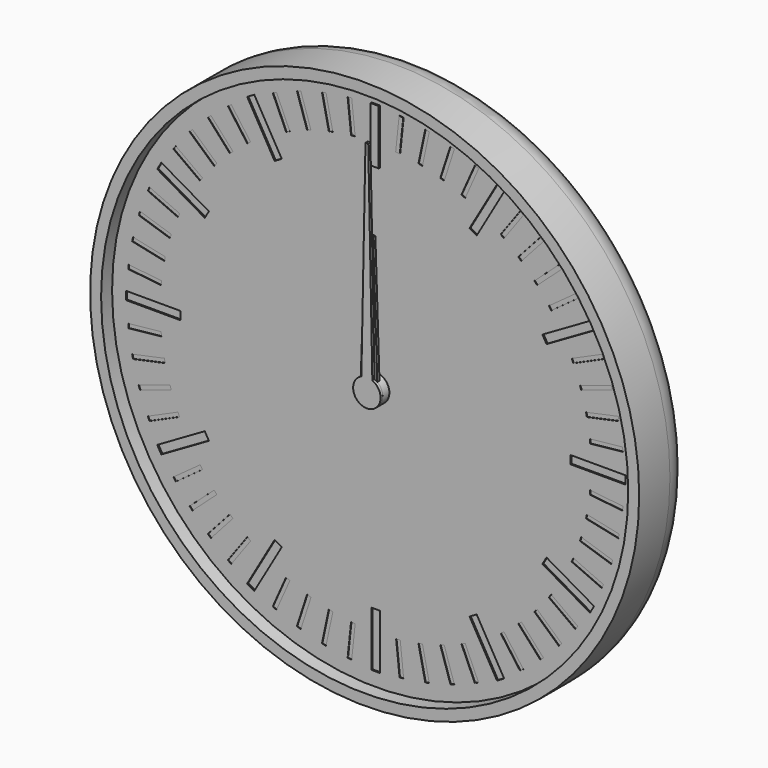
from build123d import *

# Parameters (mm, degrees)
F0_R      = 100
F1_DEPTH  = 24
F2_R      = 10
F3_T      = -4
F4_R      = 5
F4_R_2    = 3
F5_DEPTH  = 2
F6_DEPTH  = 19
F7_DEPTH  = 8
F9_DEPTH  = 4
F11_DEPTH = 4
F12_R     = 5
F12_R_2   = 3
F13_DEPTH = 2
F14_R     = 3
F15_DEPTH = 4
F17_DEPTH = 4
F18_R     = 3
F19_DEPTH = 2
F20_R     = 98
F20_R_2   = 5
F21_DEPTH = 1
F23_R     = 5
F23_R_2   = 3
F24_DEPTH = 2
F25_W     = 3
F25_H     = 20
F25_W_2   = 20
F25_H_2   = 3
F26_DEPTH = 0.5
F27_W     = 1.5
F27_H     = 12
F27_W_2   = 12
F27_H_2   = 1.5
F28_DEPTH = 0.2
F29_DEPTH = 1
F30_DEPTH = 0.4
F31_R     = 5
F31_R_2   = 3
F32_DEPTH = 5
F33_R     = 3
F34_DEPTH = 1
F36_DEPTH = 1


with BuildPart() as f1:
    # F0 (on Front) → F1 (new body)
    with BuildSketch(Plane.XZ):
        Circle(F0_R)
    extrude(amount=F1_DEPTH)

    # F2
    f2_edges = [f1.edges().sort_by_distance(p)[0] for p in [
        (-100, 0, 0),
    ]]
    fillet(f2_edges, radius=F2_R)

    # F3
    f3_openings = [f1.faces().sort_by_distance(p)[0] for p in [
        (0, -24, 0),
    ]]
    offset(amount=F3_T, openings=f3_openings)

    # F4 (on face) → F5 (join)
    with BuildSketch(Plane.XZ.offset(4)):
        Circle(F4_R)
        Circle(F4_R_2, mode=Mode.SUBTRACT)
        with Locations((40, 0)):
            Circle(F4_R)
        with Locations((40, 0)):
            Circle(F4_R_2, mode=Mode.SUBTRACT)
    extrude(amount=F5_DEPTH)


with BuildPart() as f6:
    # F6 (new): a face of the model
    f6_faces = [f1.part.faces().sort_by_distance(p)[0] for p in [
        (0, -4, 0),
    ]]
    extrude(f6_faces, amount=F6_DEPTH)

    # F8 (on face) → F9 (join)
    with BuildSketch(Plane.XZ.offset(6)):
        with BuildLine():
            ThreePointArc((9.2729637667, -1.3794085621), (9.3494561423, -0.6915886375), (9.375, 0))
            ThreePointArc((9.375, 0), (9.3494561423, 0.6915886375), (9.2729637667, 1.3794085621))
            ThreePointArc((9.2729637667, 1.3794085621), (8.9161548403, 2.8970343223), (8.3127812852, 4.3345463782))
            ThreePointArc((8.3127812852, 4.3345463782), (7.5845343223, 5.5104867402), (6.6911892658, 6.566476316))
            ThreePointArc((6.6911892658, 6.566476316), (5.5104867402, 7.5845343223), (4.1773988938, 8.3928519278))
            ThreePointArc((4.1773988938, 8.3928519278), (2.8970343223, 8.9161548403), (1.5536078905, 9.2453733036))
            ThreePointArc((1.5536078905, 9.2453733036), (0, 9.375), (-1.5536078905, 9.2453733036))
            ThreePointArc((-1.5536078905, 9.2453733036), (-2.8970343223, 8.9161548403), (-4.1773988938, 8.3928519278))
            ThreePointArc((-4.1773988938, 8.3928519278), (-5.5104867402, 7.5845343223), (-6.6911892658, 6.566476316))
            ThreePointArc((-6.6911892658, 6.566476316), (-7.5845343223, 5.5104867402), (-8.3127812852, 4.3345463782))
            ThreePointArc((-8.3127812852, 4.3345463782), (-8.9161548403, 2.8970343223), (-9.2729637667, 1.3794085621))
            ThreePointArc((-9.2729637667, 1.3794085621), (-9.375, 0), (-9.2729637667, -1.3794085621))
            ThreePointArc((-9.2729637667, -1.3794085621), (-8.9161548403, -2.8970343223), (-8.3127812852, -4.3345463782))
            ThreePointArc((-8.3127812852, -4.3345463782), (-7.5845343223, -5.5104867402), (-6.6911892658, -6.566476316))
            ThreePointArc((-6.6911892658, -6.566476316), (-5.5104867402, -7.5845343223), (-4.1773988938, -8.3928519278))
            ThreePointArc((-4.1773988938, -8.3928519278), (-2.8970343223, -8.9161548403), (-1.5536078905, -9.2453733036))
            ThreePointArc((-1.5536078905, -9.2453733036), (0, -9.375), (1.5536078905, -9.2453733036))
            ThreePointArc((1.5536078905, -9.2453733036), (2.8970343223, -8.9161548403), (4.1773988938, -8.3928519278))
            ThreePointArc((4.1773988938, -8.3928519278), (5.5104867402, -7.5845343223), (6.6911892658, -6.566476316))
            ThreePointArc((6.6911892658, -6.566476316), (7.5845343223, -5.5104867402), (8.3127812852, -4.3345463782))
            ThreePointArc((8.3127812852, -4.3345463782), (8.9161548403, -2.8970343223), (9.2729637667, -1.3794085621))
        make_face()
        with BuildLine():
            ThreePointArc((8.3127812852, 4.3345463782), (8.9161548403, 2.8970343223), (9.2729637667, 1.3794085621))
            Line((9.2729637667, 1.3794085621), (11.1823199426, 2.3946312492))
            Line((11.1823199426, 2.3946312492), (10.8182678729, 3.515068311))
            Line((10.8182678729, 3.515068311), (10.4542158031, 4.6355053728))
            Line((10.4542158031, 4.6355053728), (8.3127812852, 4.3345463782))
        make_face()
        with BuildLine():
            Line((11.1823199426, -2.3946312492), (9.2729637667, -1.3794085621))
            ThreePointArc((9.2729637667, -1.3794085621), (8.9161548403, -2.8970343223), (8.3127812852, -4.3345463782))
            Line((8.3127812852, -4.3345463782), (10.4542158031, -4.6355053728))
            Line((10.4542158031, -4.6355053728), (10.8182678729, -3.515068311))
            Line((10.8182678729, -3.515068311), (11.1823199426, -2.3946312492))
        make_face()
        with BuildLine():
            ThreePointArc((4.1773988938, 8.3928519278), (5.5104867402, 7.5845343223), (6.6911892658, 6.566476316))
            Line((6.6911892658, 6.566476316), (7.6391579371, 8.5101001246))
            Line((7.6391579371, 8.5101001246), (6.6860572448, 9.202568311))
            Line((6.6860572448, 9.202568311), (5.7329565525, 9.8950364974))
            Line((5.7329565525, 9.8950364974), (4.1773988938, 8.3928519278))
        make_face()
        with BuildLine():
            Line((7.6391579371, -8.5101001246), (6.6911892658, -6.566476316))
            ThreePointArc((6.6911892658, -6.566476316), (5.5104867402, -7.5845343223), (4.1773988938, -8.3928519278))
            Line((4.1773988938, -8.3928519278), (5.7329565525, -9.8950364974))
            Line((5.7329565525, -9.8950364974), (6.6860572448, -9.202568311))
            Line((6.6860572448, -9.202568311), (7.6391579371, -8.5101001246))
        make_face()
        with BuildLine():
            ThreePointArc((-1.5536078905, 9.2453733036), (0, 9.375), (1.5536078905, 9.2453733036))
            Line((1.5536078905, 9.2453733036), (1.1780972451, 11.375))
            Line((1.1780972451, 11.375), (0, 11.375))
            Line((0, 11.375), (-1.1780972451, 11.375))
            Line((-1.1780972451, 11.375), (-1.5536078905, 9.2453733036))
        make_face()
        with BuildLine():
            Line((1.1780972451, -11.375), (1.5536078905, -9.2453733036))
            ThreePointArc((1.5536078905, -9.2453733036), (0, -9.375), (-1.5536078905, -9.2453733036))
            Line((-1.5536078905, -9.2453733036), (-1.1780972451, -11.375))
            Line((-1.1780972451, -11.375), (0, -11.375))
            Line((0, -11.375), (1.1780972451, -11.375))
        make_face()
        with BuildLine():
            ThreePointArc((-6.6911892658, 6.566476316), (-5.5104867402, 7.5845343223), (-4.1773988938, 8.3928519278))
            Line((-4.1773988938, 8.3928519278), (-5.7329565525, 9.8950364974))
            Line((-5.7329565525, 9.8950364974), (-6.6860572448, 9.202568311))
            Line((-6.6860572448, 9.202568311), (-7.6391579371, 8.5101001246))
            Line((-7.6391579371, 8.5101001246), (-6.6911892658, 6.566476316))
        make_face()
        with BuildLine():
            Line((-5.7329565525, -9.8950364974), (-4.1773988938, -8.3928519278))
            ThreePointArc((-4.1773988938, -8.3928519278), (-5.5104867402, -7.5845343223), (-6.6911892658, -6.566476316))
            Line((-6.6911892658, -6.566476316), (-7.6391579371, -8.5101001246))
            Line((-7.6391579371, -8.5101001246), (-6.6860572448, -9.202568311))
            Line((-6.6860572448, -9.202568311), (-5.7329565525, -9.8950364974))
        make_face()
        with BuildLine():
            ThreePointArc((-9.2729637667, 1.3794085621), (-8.9161548403, 2.8970343223), (-8.3127812852, 4.3345463782))
            Line((-8.3127812852, 4.3345463782), (-10.4542158031, 4.6355053728))
            Line((-10.4542158031, 4.6355053728), (-10.8182678729, 3.515068311))
            Line((-10.8182678729, 3.515068311), (-11.1823199426, 2.3946312492))
            Line((-11.1823199426, 2.3946312492), (-9.2729637667, 1.3794085621))
        make_face()
        with BuildLine():
            Line((-10.4542158031, -4.6355053728), (-8.3127812852, -4.3345463782))
            ThreePointArc((-8.3127812852, -4.3345463782), (-8.9161548403, -2.8970343223), (-9.2729637667, -1.3794085621))
            Line((-9.2729637667, -1.3794085621), (-11.1823199426, -2.3946312492))
            Line((-11.1823199426, -2.3946312492), (-10.8182678729, -3.515068311))
            Line((-10.8182678729, -3.515068311), (-10.4542158031, -4.6355053728))
        make_face()
    extrude(amount=F9_DEPTH)

    # F35 (on face) → F36 (join)
    with BuildSketch(Plane.XZ.offset(23)):
        with BuildLine():
            ThreePointArc((-2, 4.582575695), (-2.7386127875, -4.1833001327), (5, 0))
            ThreePointArc((5, 0), (4.1833001327, 2.7386127875), (2, 4.582575695))
            ThreePointArc((2, 4.582575695), (0, 5), (-2, 4.582575695))
        make_face()
        with BuildLine():
            ThreePointArc((-2, 4.582575695), (0, 5), (2, 4.582575695))
            Line((2, 4.582575695), (0.5, 80))
            Line((0.5, 80), (0, 80))
            Line((0, 80), (-0.5, 80))
            Line((-0.5, 80), (-2, 4.582575695))
        make_face()
    extrude(amount=-F36_DEPTH)


with BuildPart() as f7:
    # F7 (new): a face of the model
    f7_faces = [f1.part.faces().sort_by_distance(p)[0] for p in [
        (40, -4, 0),
    ]]
    extrude(f7_faces, amount=F7_DEPTH)

    # F10 (on face) → F11 (join)
    with BuildSketch(Plane.XZ.offset(6)):
        with BuildLine():
            ThreePointArc((68.0829066802, -1.5381733945), (68.1144747006, -0.7693746225), (68.125, 0))
            ThreePointArc((68.125, 0), (68.1144747006, 0.7693746225), (68.0829066802, 1.5381733945))
            ThreePointArc((68.0829066802, 1.5381733945), (67.9709283072, 2.9398630294), (67.7890320221, 4.3342039956))
            ThreePointArc((67.7890320221, 4.3342039956), (67.5104012706, 5.8475163042), (67.1494235596, 7.3433252263))
            ThreePointArc((67.1494235596, 7.3433252263), (66.7484645208, 8.6911029668), (66.280643318, 10.0171558733))
            ThreePointArc((66.280643318, 10.0171558733), (65.6934659962, 11.4394680865), (65.0293803521, 12.8275385085))
            ThreePointArc((65.0293803521, 12.8275385085), (64.3569644814, 14.0625), (63.6236643925, 15.2623099717))
            ThreePointArc((63.6236643925, 15.2623099717), (62.7536029668, 16.5314602207), (61.815433119, 17.7511268046))
            ThreePointArc((61.815433119, 17.7511268046), (60.9009482166, 18.8192983038), (59.934217974, 19.8404278876))
            ThreePointArc((59.934217974, 19.8404278876), (58.8192983038, 20.9009482166), (57.6480467764, 21.8989056799))
            ThreePointArc((57.6480467764, 21.8989056799), (56.5314602207, 22.7536029668), (55.3735505752, 23.5514238999))
            ThreePointArc((55.3735505752, 23.5514238999), (54.0625, 24.3569644814), (52.709356105, 25.0895972944))
            ThreePointArc((52.709356105, 25.0895972944), (51.4394680865, 25.6934659962), (50.1409852457, 26.2331096755))
            ThreePointArc((50.1409852457, 26.2331096755), (48.6911029668, 26.7484645208), (47.2152055856, 27.1837531139))
            ThreePointArc((47.2152055856, 27.1837531139), (45.8475163042, 27.5104012706), (44.4652101991, 27.7682826779))
            ThreePointArc((44.4652101991, 27.7682826779), (42.9398630294, 27.9709283072), (41.4057159597, 28.0898484802))
            ThreePointArc((41.4057159597, 28.0898484802), (40, 28.125), (38.5942840403, 28.0898484802))
            ThreePointArc((38.5942840403, 28.0898484802), (37.0601369706, 27.9709283072), (35.5347898009, 27.7682826779))
            ThreePointArc((35.5347898009, 27.7682826779), (34.1524836958, 27.5104012706), (32.7847944144, 27.1837531139))
            ThreePointArc((32.7847944144, 27.1837531139), (31.3088970332, 26.7484645208), (29.8590147543, 26.2331096755))
            ThreePointArc((29.8590147543, 26.2331096755), (28.5605319135, 25.6934659962), (27.290643895, 25.0895972944))
            ThreePointArc((27.290643895, 25.0895972944), (25.9375, 24.3569644814), (24.6264494248, 23.5514238999))
            ThreePointArc((24.6264494248, 23.5514238999), (23.4685397793, 22.7536029668), (22.3519532236, 21.8989056799))
            ThreePointArc((22.3519532236, 21.8989056799), (21.1807016962, 20.9009482166), (20.065782026, 19.8404278876))
            ThreePointArc((20.065782026, 19.8404278876), (19.0990517834, 18.8192983038), (18.184566881, 17.7511268046))
            ThreePointArc((18.184566881, 17.7511268046), (17.2463970332, 16.5314602207), (16.3763356075, 15.2623099717))
            ThreePointArc((16.3763356075, 15.2623099717), (15.6430355186, 14.0625), (14.9706196479, 12.8275385085))
            ThreePointArc((14.9706196479, 12.8275385085), (14.3065340038, 11.4394680865), (13.719356682, 10.0171558733))
            ThreePointArc((13.719356682, 10.0171558733), (13.2515354792, 8.6911029668), (12.8505764404, 7.3433252263))
            ThreePointArc((12.8505764404, 7.3433252263), (12.4895987294, 5.8475163042), (12.2109679779, 4.3342039956))
            ThreePointArc((12.2109679779, 4.3342039956), (12.0290716928, 2.9398630294), (11.9170933198, 1.5381733945))
            ThreePointArc((11.9170933198, 1.5381733945), (11.875, 0), (11.9170933198, -1.5381733945))
            ThreePointArc((11.9170933198, -1.5381733945), (12.0290716928, -2.9398630294), (12.2109679779, -4.3342039956))
            ThreePointArc((12.2109679779, -4.3342039956), (12.4895987294, -5.8475163042), (12.8505764404, -7.3433252263))
            ThreePointArc((12.8505764404, -7.3433252263), (13.2515354792, -8.6911029668), (13.719356682, -10.0171558733))
            ThreePointArc((13.719356682, -10.0171558733), (14.3065340038, -11.4394680865), (14.9706196479, -12.8275385085))
            ThreePointArc((14.9706196479, -12.8275385085), (15.6430355186, -14.0625), (16.3763356075, -15.2623099717))
            ThreePointArc((16.3763356075, -15.2623099717), (17.2463970332, -16.5314602207), (18.184566881, -17.7511268046))
            ThreePointArc((18.184566881, -17.7511268046), (19.0990517834, -18.8192983038), (20.065782026, -19.8404278876))
            ThreePointArc((20.065782026, -19.8404278876), (21.1807016962, -20.9009482166), (22.3519532236, -21.8989056799))
            ThreePointArc((22.3519532236, -21.8989056799), (23.4685397793, -22.7536029668), (24.6264494248, -23.5514238999))
            ThreePointArc((24.6264494248, -23.5514238999), (25.9375, -24.3569644814), (27.290643895, -25.0895972944))
            ThreePointArc((27.290643895, -25.0895972944), (28.5605319135, -25.6934659962), (29.8590147543, -26.2331096755))
            ThreePointArc((29.8590147543, -26.2331096755), (31.3088970332, -26.7484645208), (32.7847944144, -27.1837531139))
            ThreePointArc((32.7847944144, -27.1837531139), (34.1524836958, -27.5104012706), (35.5347898009, -27.7682826779))
            ThreePointArc((35.5347898009, -27.7682826779), (37.0601369706, -27.9709283072), (38.5942840403, -28.0898484802))
            ThreePointArc((38.5942840403, -28.0898484802), (40, -28.125), (41.4057159597, -28.0898484802))
            ThreePointArc((41.4057159597, -28.0898484802), (42.9398630294, -27.9709283072), (44.4652101991, -27.7682826779))
            ThreePointArc((44.4652101991, -27.7682826779), (45.8475163042, -27.5104012706), (47.2152055856, -27.1837531139))
            ThreePointArc((47.2152055856, -27.1837531139), (48.6911029668, -26.7484645208), (50.1409852457, -26.2331096755))
            ThreePointArc((50.1409852457, -26.2331096755), (51.4394680865, -25.6934659962), (52.709356105, -25.0895972944))
            ThreePointArc((52.709356105, -25.0895972944), (54.0625, -24.3569644814), (55.3735505752, -23.5514238999))
            ThreePointArc((55.3735505752, -23.5514238999), (56.5314602207, -22.7536029668), (57.6480467764, -21.8989056799))
            ThreePointArc((57.6480467764, -21.8989056799), (58.8192983038, -20.9009482166), (59.934217974, -19.8404278876))
            ThreePointArc((59.934217974, -19.8404278876), (60.9009482166, -18.8192983038), (61.815433119, -17.7511268046))
            ThreePointArc((61.815433119, -17.7511268046), (62.7536029668, -16.5314602207), (63.6236643925, -15.2623099717))
            ThreePointArc((63.6236643925, -15.2623099717), (64.3569644814, -14.0625), (65.0293803521, -12.8275385085))
            ThreePointArc((65.0293803521, -12.8275385085), (65.6934659962, -11.4394680865), (66.280643318, -10.0171558733))
            ThreePointArc((66.280643318, -10.0171558733), (66.7484645208, -8.6911029668), (67.1494235596, -7.3433252263))
            ThreePointArc((67.1494235596, -7.3433252263), (67.5104012706, -5.8475163042), (67.7890320221, -4.3342039956))
            ThreePointArc((67.7890320221, -4.3342039956), (67.9709283072, -2.9398630294), (68.0829066802, -1.5381733945))
        make_face()
        with BuildLine():
            ThreePointArc((68.0829066802, 1.5381733945), (68.1144747006, 0.7693746225), (68.125, 0))
            ThreePointArc((68.125, 0), (68.1144747006, -0.7693746225), (68.0829066802, -1.5381733945))
            Line((68.0829066802, -1.5381733945), (70.125, -1.1780972451))
            Line((70.125, -1.1780972451), (70.125, 0))
            Line((70.125, 0), (70.125, 1.1780972451))
            Line((70.125, 1.1780972451), (68.0829066802, 1.5381733945))
        make_face()
        with BuildLine():
            ThreePointArc((67.1494235596, 7.3433252263), (67.5104012706, 5.8475163042), (67.7890320221, 4.3342039956))
            Line((67.7890320221, 4.3342039956), (69.7116366623, 5.1109866922))
            Line((69.7116366623, 5.1109866922), (69.4666964721, 6.2633396859))
            Line((69.4666964721, 6.2633396859), (69.2217562819, 7.4156926796))
            Line((69.2217562819, 7.4156926796), (67.1494235596, 7.3433252263))
        make_face()
        with BuildLine():
            Line((69.7116366623, -5.1109866922), (67.7890320221, -4.3342039956))
            ThreePointArc((67.7890320221, -4.3342039956), (67.5104012706, -5.8475163042), (67.1494235596, -7.3433252263))
            Line((67.1494235596, -7.3433252263), (69.2217562819, -7.4156926796))
            Line((69.2217562819, -7.4156926796), (69.4666964721, -6.2633396859))
            Line((69.4666964721, -6.2633396859), (69.7116366623, -5.1109866922))
        make_face()
        with BuildLine():
            ThreePointArc((65.0293803521, 12.8275385085), (65.6934659962, 11.4394680865), (66.280643318, 10.0171558733))
            Line((66.280643318, 10.0171558733), (67.9997322302, 11.1766959857))
            Line((67.9997322302, 11.1766959857), (67.5205569115, 12.2529413727))
            Line((67.5205569115, 12.2529413727), (67.0413815928, 13.3291867596))
            Line((67.0413815928, 13.3291867596), (65.0293803521, 12.8275385085))
        make_face()
        with BuildLine():
            Line((67.9997322302, -11.1766959857), (66.280643318, -10.0171558733))
            ThreePointArc((66.280643318, -10.0171558733), (65.6934659962, -11.4394680865), (65.0293803521, -12.8275385085))
            Line((65.0293803521, -12.8275385085), (67.0413815928, -13.3291867596))
            Line((67.0413815928, -13.3291867596), (67.5205569115, -12.2529413727))
            Line((67.5205569115, -12.2529413727), (67.9997322302, -11.1766959857))
        make_face()
        with BuildLine():
            ThreePointArc((61.815433119, 17.7511268046), (62.7536029668, 16.5314602207), (63.6236643925, 15.2623099717))
            Line((63.6236643925, 15.2623099717), (65.064105142, 16.753930033))
            Line((65.064105142, 16.753930033), (64.3716369555, 17.7070307253))
            Line((64.3716369555, 17.7070307253), (63.6791687691, 18.6601314176))
            Line((63.6791687691, 18.6601314176), (61.815433119, 17.7511268046))
        make_face()
        with BuildLine():
            Line((65.064105142, -16.753930033), (63.6236643925, -15.2623099717))
            ThreePointArc((63.6236643925, -15.2623099717), (62.7536029668, -16.5314602207), (61.815433119, -17.7511268046))
            Line((61.815433119, -17.7511268046), (63.6791687691, -18.6601314176))
            Line((63.6791687691, -18.6601314176), (64.3716369555, -17.7070307253))
            Line((64.3716369555, -17.7070307253), (65.064105142, -16.753930033))
        make_face()
        with BuildLine():
            ThreePointArc((57.6480467764, 21.8989056799), (58.8192983038, 20.9009482166), (59.934217974, 19.8404278876))
            Line((59.934217974, 19.8404278876), (61.0330563882, 21.5989369435))
            Line((61.0330563882, 21.5989369435), (60.1575595166, 22.3872378675))
            Line((60.1575595166, 22.3872378675), (59.282062645, 23.1755387915))
            Line((59.282062645, 23.1755387915), (57.6480467764, 21.8989056799))
        make_face()
        with BuildLine():
            Line((61.0330563882, -21.5989369435), (59.934217974, -19.8404278876))
            ThreePointArc((59.934217974, -19.8404278876), (58.8192983038, -20.9009482166), (57.6480467764, -21.8989056799))
            Line((57.6480467764, -21.8989056799), (59.282062645, -23.1755387915))
            Line((59.282062645, -23.1755387915), (60.1575595166, -22.3872378675))
            Line((60.1575595166, -22.3872378675), (61.0330563882, -21.5989369435))
        make_face()
        with BuildLine():
            ThreePointArc((52.709356105, 25.0895972944), (54.0625, 24.3569644814), (55.3735505752, 23.5514238999))
            Line((55.3735505752, 23.5514238999), (56.0827621424, 25.4999666665))
            Line((56.0827621424, 25.4999666665), (55.0625, 26.089015289))
            Line((55.0625, 26.089015289), (54.0422378576, 26.6780639116))
            Line((54.0422378576, 26.6780639116), (52.709356105, 25.0895972944))
        make_face()
        with BuildLine():
            Line((56.0827621424, -25.4999666665), (55.3735505752, -23.5514238999))
            ThreePointArc((55.3735505752, -23.5514238999), (54.0625, -24.3569644814), (52.709356105, -25.0895972944))
            Line((52.709356105, -25.0895972944), (54.0422378576, -26.6780639116))
            Line((54.0422378576, -26.6780639116), (55.0625, -26.089015289))
            Line((55.0625, -26.089015289), (56.0827621424, -25.4999666665))
        make_face()
        with BuildLine():
            ThreePointArc((47.2152055856, 27.1837531139), (48.6911029668, 26.7484645208), (50.1409852457, 26.2331096755))
            Line((50.1409852457, 26.2331096755), (50.4295740173, 28.2865254836))
            Line((50.4295740173, 28.2865254836), (49.3091369555, 28.6505775534))
            Line((49.3091369555, 28.6505775534), (48.1886998938, 29.0146296232))
            Line((48.1886998938, 29.0146296232), (47.2152055856, 27.1837531139))
        make_face()
        with BuildLine():
            Line((50.4295740173, -28.2865254836), (50.1409852457, -26.2331096755))
            ThreePointArc((50.1409852457, -26.2331096755), (48.6911029668, -26.7484645208), (47.2152055856, -27.1837531139))
            Line((47.2152055856, -27.1837531139), (48.1886998938, -29.0146296232))
            Line((48.1886998938, -29.0146296232), (49.3091369555, -28.6505775534))
            Line((49.3091369555, -28.6505775534), (50.4295740173, -28.2865254836))
        make_face()
        with BuildLine():
            ThreePointArc((41.4057159597, 28.0898484802), (42.9398630294, 27.9709283072), (44.4652101991, 27.7682826779))
            Line((44.4652101991, 27.7682826779), (44.3205634611, 29.8368274034))
            Line((44.3205634611, 29.8368274034), (43.1489199559, 29.959972098))
            Line((43.1489199559, 29.959972098), (41.9772764508, 30.0831167926))
            Line((41.9772764508, 30.0831167926), (41.4057159597, 28.0898484802))
        make_face()
        with BuildLine():
            Line((44.3205634611, -29.8368274034), (44.4652101991, -27.7682826779))
            ThreePointArc((44.4652101991, -27.7682826779), (42.9398630294, -27.9709283072), (41.4057159597, -28.0898484802))
            Line((41.4057159597, -28.0898484802), (41.9772764508, -30.0831167926))
            Line((41.9772764508, -30.0831167926), (43.1489199559, -29.959972098))
            Line((43.1489199559, -29.959972098), (44.3205634611, -29.8368274034))
        make_face()
        with BuildLine():
            ThreePointArc((35.5347898009, 27.7682826779), (37.0601369706, 27.9709283072), (38.5942840403, 28.0898484802))
            Line((38.5942840403, 28.0898484802), (38.0227235492, 30.0831167926))
            Line((38.0227235492, 30.0831167926), (36.8510800441, 29.959972098))
            Line((36.8510800441, 29.959972098), (35.6794365389, 29.8368274034))
            Line((35.6794365389, 29.8368274034), (35.5347898009, 27.7682826779))
        make_face()
        with BuildLine():
            Line((38.0227235492, -30.0831167926), (38.5942840403, -28.0898484802))
            ThreePointArc((38.5942840403, -28.0898484802), (37.0601369706, -27.9709283072), (35.5347898009, -27.7682826779))
            Line((35.5347898009, -27.7682826779), (35.6794365389, -29.8368274034))
            Line((35.6794365389, -29.8368274034), (36.8510800441, -29.959972098))
            Line((36.8510800441, -29.959972098), (38.0227235492, -30.0831167926))
        make_face()
        with BuildLine():
            ThreePointArc((29.8590147543, 26.2331096755), (31.3088970332, 26.7484645208), (32.7847944144, 27.1837531139))
            Line((32.7847944144, 27.1837531139), (31.8113001062, 29.0146296232))
            Line((31.8113001062, 29.0146296232), (30.6908630445, 28.6505775534))
            Line((30.6908630445, 28.6505775534), (29.5704259827, 28.2865254836))
            Line((29.5704259827, 28.2865254836), (29.8590147543, 26.2331096755))
        make_face()
        with BuildLine():
            Line((31.8113001062, -29.0146296232), (32.7847944144, -27.1837531139))
            ThreePointArc((32.7847944144, -27.1837531139), (31.3088970332, -26.7484645208), (29.8590147543, -26.2331096755))
            Line((29.8590147543, -26.2331096755), (29.5704259827, -28.2865254836))
            Line((29.5704259827, -28.2865254836), (30.6908630445, -28.6505775534))
            Line((30.6908630445, -28.6505775534), (31.8113001062, -29.0146296232))
        make_face()
        with BuildLine():
            ThreePointArc((24.6264494248, 23.5514238999), (25.9375, 24.3569644814), (27.290643895, 25.0895972944))
            Line((27.290643895, 25.0895972944), (25.9577621424, 26.6780639116))
            Line((25.9577621424, 26.6780639116), (24.9375, 26.089015289))
            Line((24.9375, 26.089015289), (23.9172378576, 25.4999666665))
            Line((23.9172378576, 25.4999666665), (24.6264494248, 23.5514238999))
        make_face()
        with BuildLine():
            Line((25.9577621424, -26.6780639116), (27.290643895, -25.0895972944))
            ThreePointArc((27.290643895, -25.0895972944), (25.9375, -24.3569644814), (24.6264494248, -23.5514238999))
            Line((24.6264494248, -23.5514238999), (23.9172378576, -25.4999666665))
            Line((23.9172378576, -25.4999666665), (24.9375, -26.089015289))
            Line((24.9375, -26.089015289), (25.9577621424, -26.6780639116))
        make_face()
        with BuildLine():
            ThreePointArc((20.065782026, 19.8404278876), (21.1807016962, 20.9009482166), (22.3519532236, 21.8989056799))
            Line((22.3519532236, 21.8989056799), (20.717937355, 23.1755387915))
            Line((20.717937355, 23.1755387915), (19.8424404834, 22.3872378675))
            Line((19.8424404834, 22.3872378675), (18.9669436118, 21.5989369435))
            Line((18.9669436118, 21.5989369435), (20.065782026, 19.8404278876))
        make_face()
        with BuildLine():
            Line((20.717937355, -23.1755387915), (22.3519532236, -21.8989056799))
            ThreePointArc((22.3519532236, -21.8989056799), (21.1807016962, -20.9009482166), (20.065782026, -19.8404278876))
            Line((20.065782026, -19.8404278876), (18.9669436118, -21.5989369435))
            Line((18.9669436118, -21.5989369435), (19.8424404834, -22.3872378675))
            Line((19.8424404834, -22.3872378675), (20.717937355, -23.1755387915))
        make_face()
        with BuildLine():
            ThreePointArc((16.3763356075, 15.2623099717), (17.2463970332, 16.5314602207), (18.184566881, 17.7511268046))
            Line((18.184566881, 17.7511268046), (16.3208312309, 18.6601314176))
            Line((16.3208312309, 18.6601314176), (15.6283630445, 17.7070307253))
            Line((15.6283630445, 17.7070307253), (14.935894858, 16.753930033))
            Line((14.935894858, 16.753930033), (16.3763356075, 15.2623099717))
        make_face()
        with BuildLine():
            Line((16.3208312309, -18.6601314176), (18.184566881, -17.7511268046))
            ThreePointArc((18.184566881, -17.7511268046), (17.2463970332, -16.5314602207), (16.3763356075, -15.2623099717))
            Line((16.3763356075, -15.2623099717), (14.935894858, -16.753930033))
            Line((14.935894858, -16.753930033), (15.6283630445, -17.7070307253))
            Line((15.6283630445, -17.7070307253), (16.3208312309, -18.6601314176))
        make_face()
        with BuildLine():
            ThreePointArc((13.719356682, 10.0171558733), (14.3065340038, 11.4394680865), (14.9706196479, 12.8275385085))
            Line((14.9706196479, 12.8275385085), (12.9586184072, 13.3291867596))
            Line((12.9586184072, 13.3291867596), (12.4794430885, 12.2529413727))
            Line((12.4794430885, 12.2529413727), (12.0002677698, 11.1766959857))
            Line((12.0002677698, 11.1766959857), (13.719356682, 10.0171558733))
        make_face()
        with BuildLine():
            Line((12.9586184072, -13.3291867596), (14.9706196479, -12.8275385085))
            ThreePointArc((14.9706196479, -12.8275385085), (14.3065340038, -11.4394680865), (13.719356682, -10.0171558733))
            Line((13.719356682, -10.0171558733), (12.0002677698, -11.1766959857))
            Line((12.0002677698, -11.1766959857), (12.4794430885, -12.2529413727))
            Line((12.4794430885, -12.2529413727), (12.9586184072, -13.3291867596))
        make_face()
        with BuildLine():
            ThreePointArc((12.2109679779, 4.3342039956), (12.4895987294, 5.8475163042), (12.8505764404, 7.3433252263))
            Line((12.8505764404, 7.3433252263), (10.7782437181, 7.4156926796))
            Line((10.7782437181, 7.4156926796), (10.5333035279, 6.2633396859))
            Line((10.5333035279, 6.2633396859), (10.2883633377, 5.1109866922))
            Line((10.2883633377, 5.1109866922), (12.2109679779, 4.3342039956))
        make_face()
        with BuildLine():
            Line((10.7782437181, -7.4156926796), (12.8505764404, -7.3433252263))
            ThreePointArc((12.8505764404, -7.3433252263), (12.4895987294, -5.8475163042), (12.2109679779, -4.3342039956))
            Line((12.2109679779, -4.3342039956), (10.2883633377, -5.1109866922))
            Line((10.2883633377, -5.1109866922), (10.5333035279, -6.2633396859))
            Line((10.5333035279, -6.2633396859), (10.7782437181, -7.4156926796))
        make_face()
        with BuildLine():
            ThreePointArc((11.9170933198, -1.5381733945), (11.875, 0), (11.9170933198, 1.5381733945))
            Line((11.9170933198, 1.5381733945), (9.875, 1.1780972451))
            Line((9.875, 1.1780972451), (9.875, 0))
            Line((9.875, 0), (9.875, -1.1780972451))
            Line((9.875, -1.1780972451), (11.9170933198, -1.5381733945))
        make_face()
    extrude(amount=F11_DEPTH)

    # F16 (on face) → F17 (join)
    with BuildSketch(Plane.XZ.offset(12)):
        with BuildLine():
            ThreePointArc((47.4288750323, -1.0304444454), (47.4821976298, -0.5164480894), (47.5, 0))
            ThreePointArc((47.5, 0), (47.4821976298, 0.5164480894), (47.4288750323, 1.0304444454))
            ThreePointArc((47.4288750323, 1.0304444454), (47.1329238722, 2.3176274578), (46.6157661985, 3.532936117))
            ThreePointArc((46.6157661985, 3.532936117), (46.0676274578, 4.4083893922), (45.4044061018, 5.2002302532))
            ThreePointArc((45.4044061018, 5.2002302532), (44.4083893922, 6.0676274578), (43.2756595386, 6.7468551628))
            ThreePointArc((43.2756595386, 6.7468551628), (42.3176274578, 7.1329238722), (41.3156377295, 7.3837048536))
            ThreePointArc((41.3156377295, 7.3837048536), (40, 7.5), (38.6843622705, 7.3837048536))
            ThreePointArc((38.6843622705, 7.3837048536), (37.6823725422, 7.1329238722), (36.7243404614, 6.7468551628))
            ThreePointArc((36.7243404614, 6.7468551628), (35.5916106078, 6.0676274578), (34.5955938982, 5.2002302532))
            ThreePointArc((34.5955938982, 5.2002302532), (33.9323725422, 4.4083893922), (33.3842338015, 3.532936117))
            ThreePointArc((33.3842338015, 3.532936117), (32.8670761278, 2.3176274578), (32.5711249677, 1.0304444454))
            ThreePointArc((32.5711249677, 1.0304444454), (32.5, 0), (32.5711249677, -1.0304444454))
            ThreePointArc((32.5711249677, -1.0304444454), (32.8670761278, -2.3176274578), (33.3842338015, -3.532936117))
            ThreePointArc((33.3842338015, -3.532936117), (33.9323725422, -4.4083893922), (34.5955938982, -5.2002302532))
            ThreePointArc((34.5955938982, -5.2002302532), (35.5916106078, -6.0676274578), (36.7243404614, -6.7468551628))
            ThreePointArc((36.7243404614, -6.7468551628), (37.6823725422, -7.1329238722), (38.6843622705, -7.3837048536))
            ThreePointArc((38.6843622705, -7.3837048536), (40, -7.5), (41.3156377295, -7.3837048536))
            ThreePointArc((41.3156377295, -7.3837048536), (42.3176274578, -7.1329238722), (43.2756595386, -6.7468551628))
            ThreePointArc((43.2756595386, -6.7468551628), (44.4083893922, -6.0676274578), (45.4044061018, -5.2002302532))
            ThreePointArc((45.4044061018, -5.2002302532), (46.0676274578, -4.4083893922), (46.6157661985, -3.532936117))
            ThreePointArc((46.6157661985, -3.532936117), (47.1329238722, -2.3176274578), (47.4288750323, -1.0304444454))
        make_face()
        with BuildLine():
            ThreePointArc((46.6157661985, 3.532936117), (47.1329238722, 2.3176274578), (47.4288750323, 1.0304444454))
            Line((47.4288750323, 1.0304444454), (49.3262785606, 2.0393117971))
            Line((49.3262785606, 2.0393117971), (48.743795249, 3.832011096))
            Line((48.743795249, 3.832011096), (46.6157661985, 3.532936117))
        make_face()
        with BuildLine():
            Line((49.3262785606, -2.0393117971), (47.4288750323, -1.0304444454))
            ThreePointArc((47.4288750323, -1.0304444454), (47.1329238722, -2.3176274578), (46.6157661985, -3.532936117))
            Line((46.6157661985, -3.532936117), (48.743795249, -3.832011096))
            Line((48.743795249, -3.832011096), (49.3262785606, -2.0393117971))
        make_face()
        with BuildLine():
            ThreePointArc((43.2756595386, 6.7468551628), (44.4083893922, 6.0676274578), (45.4044061018, 5.2002302532))
            Line((45.4044061018, 5.2002302532), (46.3464404506, 7.1316868974))
            Line((46.3464404506, 7.1316868974), (44.8214793429, 8.2396359957))
            Line((44.8214793429, 8.2396359957), (43.2756595386, 6.7468551628))
        make_face()
        with BuildLine():
            Line((46.3464404506, -7.1316868974), (45.4044061018, -5.2002302532))
            ThreePointArc((45.4044061018, -5.2002302532), (44.4083893922, -6.0676274578), (43.2756595386, -6.7468551628))
            Line((43.2756595386, -6.7468551628), (44.8214793429, -8.2396359957))
            Line((44.8214793429, -8.2396359957), (46.3464404506, -7.1316868974))
        make_face()
        with BuildLine():
            ThreePointArc((38.6843622705, 7.3837048536), (40, 7.5), (41.3156377295, 7.3837048536))
            Line((41.3156377295, 7.3837048536), (40.9424777961, 9.5))
            Line((40.9424777961, 9.5), (39.0575222039, 9.5))
            Line((39.0575222039, 9.5), (38.6843622705, 7.3837048536))
        make_face()
        with BuildLine():
            Line((40.9424777961, -9.5), (41.3156377295, -7.3837048536))
            ThreePointArc((41.3156377295, -7.3837048536), (40, -7.5), (38.6843622705, -7.3837048536))
            Line((38.6843622705, -7.3837048536), (39.0575222039, -9.5))
            Line((39.0575222039, -9.5), (40.9424777961, -9.5))
        make_face()
        with BuildLine():
            ThreePointArc((34.5955938982, 5.2002302532), (35.5916106078, 6.0676274578), (36.7243404614, 6.7468551628))
            Line((36.7243404614, 6.7468551628), (35.1785206571, 8.2396359957))
            Line((35.1785206571, 8.2396359957), (33.6535595494, 7.1316868974))
            Line((33.6535595494, 7.1316868974), (34.5955938982, 5.2002302532))
        make_face()
        with BuildLine():
            Line((35.1785206571, -8.2396359957), (36.7243404614, -6.7468551628))
            ThreePointArc((36.7243404614, -6.7468551628), (35.5916106078, -6.0676274578), (34.5955938982, -5.2002302532))
            Line((34.5955938982, -5.2002302532), (33.6535595494, -7.1316868974))
            Line((33.6535595494, -7.1316868974), (35.1785206571, -8.2396359957))
        make_face()
        with BuildLine():
            ThreePointArc((32.5711249677, 1.0304444454), (32.8670761278, 2.3176274578), (33.3842338015, 3.532936117))
            Line((33.3842338015, 3.532936117), (31.256204751, 3.832011096))
            Line((31.256204751, 3.832011096), (30.6737214394, 2.0393117971))
            Line((30.6737214394, 2.0393117971), (32.5711249677, 1.0304444454))
        make_face()
        with BuildLine():
            Line((31.256204751, -3.832011096), (33.3842338015, -3.532936117))
            ThreePointArc((33.3842338015, -3.532936117), (32.8670761278, -2.3176274578), (32.5711249677, -1.0304444454))
            Line((32.5711249677, -1.0304444454), (30.6737214394, -2.0393117971))
            Line((30.6737214394, -2.0393117971), (31.256204751, -3.832011096))
        make_face()
    extrude(amount=F17_DEPTH)

    # F18 (on face) → F19 (join)
    with BuildSketch(Plane.XZ.offset(16)):
        with Locations((40, 0)):
            Circle(F18_R)
    extrude(amount=F19_DEPTH)


with BuildPart() as f13:
    # F12 (on face) → F13 (new body)
    with BuildSketch(Plane.XZ.offset(10)):
        Circle(F12_R)
        Circle(F12_R_2, mode=Mode.SUBTRACT)
    extrude(amount=F13_DEPTH)

    # F14 (on face) → F15 (join)
    with BuildSketch(Plane.XZ.offset(12)):
        with BuildLine():
            ThreePointArc((29.9718156995, -1.3001014101), (29.9929530972, -0.6502034357), (30, 0))
            ThreePointArc((30, 0), (29.9929530972, 0.6502034357), (29.9718156995, 1.3001014101))
            ThreePointArc((29.9718156995, 1.3001014101), (29.907520012, 2.3537728718), (29.8061935814, 3.4045299509))
            ThreePointArc((29.8061935814, 3.4045299509), (29.6306502179, 4.6930339512), (29.3994322443, 5.9727199596))
            ThreePointArc((29.3994322443, 5.9727199596), (29.1710976119, 7.0033609157), (28.9066440563, 8.0253304855))
            ThreePointArc((28.9066440563, 8.0253304855), (28.5316954889, 9.2705098312), (28.1031371961, 10.4982703213))
            ThreePointArc((28.1031371961, 10.4982703213), (27.7163859753, 11.480502971), (27.2953170189, 12.448520749))
            ThreePointArc((27.2953170189, 12.448520749), (26.7301957257, 13.6197149922), (26.1148496411, 14.765318426))
            ThreePointArc((26.1148496411, 14.765318426), (25.5792049306, 15.6749569415), (25.0118886885, 16.5651871174))
            ThreePointArc((25.0118886885, 16.5651871174), (24.2705098312, 17.6335575688), (23.4835278178, 18.6687953878))
            ThreePointArc((23.4835278178, 18.6687953878), (22.812178968, 19.4834414499), (22.1125846489, 20.2739636023))
            ThreePointArc((22.1125846489, 20.2739636023), (21.2132034356, 21.2132034356), (20.2739636023, 22.1125846489))
            ThreePointArc((20.2739636023, 22.1125846489), (19.4834414499, 22.812178968), (18.6687953878, 23.4835278178))
            ThreePointArc((18.6687953878, 23.4835278178), (17.6335575688, 24.2705098312), (16.5651871174, 25.0118886885))
            ThreePointArc((16.5651871174, 25.0118886885), (15.6749569415, 25.5792049306), (14.765318426, 26.1148496411))
            ThreePointArc((14.765318426, 26.1148496411), (13.6197149922, 26.7301957257), (12.448520749, 27.2953170189))
            ThreePointArc((12.448520749, 27.2953170189), (11.480502971, 27.7163859753), (10.4982703213, 28.1031371961))
            ThreePointArc((10.4982703213, 28.1031371961), (9.2705098312, 28.5316954889), (8.0253304855, 28.9066440563))
            ThreePointArc((8.0253304855, 28.9066440563), (7.0033609157, 29.1710976119), (5.9727199596, 29.3994322443))
            ThreePointArc((5.9727199596, 29.3994322443), (4.6930339512, 29.6306502179), (3.4045299509, 29.8061935814))
            ThreePointArc((3.4045299509, 29.8061935814), (2.3537728718, 29.907520012), (1.3001014101, 29.9718156995))
            ThreePointArc((1.3001014101, 29.9718156995), (0, 30), (-1.3001014101, 29.9718156995))
            ThreePointArc((-1.3001014101, 29.9718156995), (-2.3537728718, 29.907520012), (-3.4045299509, 29.8061935814))
            ThreePointArc((-3.4045299509, 29.8061935814), (-4.6930339512, 29.6306502179), (-5.9727199596, 29.3994322443))
            ThreePointArc((-5.9727199596, 29.3994322443), (-7.0033609157, 29.1710976119), (-8.0253304855, 28.9066440563))
            ThreePointArc((-8.0253304855, 28.9066440563), (-9.2705098312, 28.5316954889), (-10.4982703213, 28.1031371961))
            ThreePointArc((-10.4982703213, 28.1031371961), (-11.480502971, 27.7163859753), (-12.448520749, 27.2953170189))
            ThreePointArc((-12.448520749, 27.2953170189), (-13.6197149922, 26.7301957257), (-14.765318426, 26.1148496411))
            ThreePointArc((-14.765318426, 26.1148496411), (-15.6749569415, 25.5792049306), (-16.5651871174, 25.0118886885))
            ThreePointArc((-16.5651871174, 25.0118886885), (-17.6335575688, 24.2705098312), (-18.6687953878, 23.4835278178))
            ThreePointArc((-18.6687953878, 23.4835278178), (-19.4834414499, 22.812178968), (-20.2739636023, 22.1125846489))
            ThreePointArc((-20.2739636023, 22.1125846489), (-21.2132034356, 21.2132034356), (-22.1125846489, 20.2739636023))
            ThreePointArc((-22.1125846489, 20.2739636023), (-22.812178968, 19.4834414499), (-23.4835278178, 18.6687953878))
            ThreePointArc((-23.4835278178, 18.6687953878), (-24.2705098312, 17.6335575688), (-25.0118886885, 16.5651871174))
            ThreePointArc((-25.0118886885, 16.5651871174), (-25.5792049306, 15.6749569415), (-26.1148496411, 14.765318426))
            ThreePointArc((-26.1148496411, 14.765318426), (-26.7301957257, 13.6197149922), (-27.2953170189, 12.448520749))
            ThreePointArc((-27.2953170189, 12.448520749), (-27.7163859753, 11.480502971), (-28.1031371961, 10.4982703213))
            ThreePointArc((-28.1031371961, 10.4982703213), (-28.5316954889, 9.2705098312), (-28.9066440563, 8.0253304855))
            ThreePointArc((-28.9066440563, 8.0253304855), (-29.1710976119, 7.0033609157), (-29.3994322443, 5.9727199596))
            ThreePointArc((-29.3994322443, 5.9727199596), (-29.6306502179, 4.6930339512), (-29.8061935814, 3.4045299509))
            ThreePointArc((-29.8061935814, 3.4045299509), (-29.907520012, 2.3537728718), (-29.9718156995, 1.3001014101))
            ThreePointArc((-29.9718156995, 1.3001014101), (-30, 0), (-29.9718156995, -1.3001014101))
            ThreePointArc((-29.9718156995, -1.3001014101), (-29.907520012, -2.3537728718), (-29.8061935814, -3.4045299509))
            ThreePointArc((-29.8061935814, -3.4045299509), (-29.6306502179, -4.6930339512), (-29.3994322443, -5.9727199596))
            ThreePointArc((-29.3994322443, -5.9727199596), (-29.1710976119, -7.0033609157), (-28.9066440563, -8.0253304855))
            ThreePointArc((-28.9066440563, -8.0253304855), (-28.5316954889, -9.2705098312), (-28.1031371961, -10.4982703213))
            ThreePointArc((-28.1031371961, -10.4982703213), (-27.7163859753, -11.480502971), (-27.2953170189, -12.448520749))
            ThreePointArc((-27.2953170189, -12.448520749), (-26.7301957257, -13.6197149922), (-26.1148496411, -14.765318426))
            ThreePointArc((-26.1148496411, -14.765318426), (-25.5792049306, -15.6749569415), (-25.0118886885, -16.5651871174))
            ThreePointArc((-25.0118886885, -16.5651871174), (-24.2705098312, -17.6335575688), (-23.4835278178, -18.6687953878))
            ThreePointArc((-23.4835278178, -18.6687953878), (-22.812178968, -19.4834414499), (-22.1125846489, -20.2739636023))
            ThreePointArc((-22.1125846489, -20.2739636023), (-21.2132034356, -21.2132034356), (-20.2739636023, -22.1125846489))
            ThreePointArc((-20.2739636023, -22.1125846489), (-19.4834414499, -22.812178968), (-18.6687953878, -23.4835278178))
            ThreePointArc((-18.6687953878, -23.4835278178), (-17.6335575688, -24.2705098312), (-16.5651871174, -25.0118886885))
            ThreePointArc((-16.5651871174, -25.0118886885), (-15.6749569415, -25.5792049306), (-14.765318426, -26.1148496411))
            ThreePointArc((-14.765318426, -26.1148496411), (-13.6197149922, -26.7301957257), (-12.448520749, -27.2953170189))
            ThreePointArc((-12.448520749, -27.2953170189), (-11.480502971, -27.7163859753), (-10.4982703213, -28.1031371961))
            ThreePointArc((-10.4982703213, -28.1031371961), (-9.2705098312, -28.5316954889), (-8.0253304855, -28.9066440563))
            ThreePointArc((-8.0253304855, -28.9066440563), (-7.0033609157, -29.1710976119), (-5.9727199596, -29.3994322443))
            ThreePointArc((-5.9727199596, -29.3994322443), (-4.6930339512, -29.6306502179), (-3.4045299509, -29.8061935814))
            ThreePointArc((-3.4045299509, -29.8061935814), (-2.3537728718, -29.907520012), (-1.3001014101, -29.9718156995))
            ThreePointArc((-1.3001014101, -29.9718156995), (0, -30), (1.3001014101, -29.9718156995))
            ThreePointArc((1.3001014101, -29.9718156995), (2.3537728718, -29.907520012), (3.4045299509, -29.8061935814))
            ThreePointArc((3.4045299509, -29.8061935814), (4.6930339512, -29.6306502179), (5.9727199596, -29.3994322443))
            ThreePointArc((5.9727199596, -29.3994322443), (7.0033609157, -29.1710976119), (8.0253304855, -28.9066440563))
            ThreePointArc((8.0253304855, -28.9066440563), (9.2705098312, -28.5316954889), (10.4982703213, -28.1031371961))
            ThreePointArc((10.4982703213, -28.1031371961), (11.480502971, -27.7163859753), (12.448520749, -27.2953170189))
            ThreePointArc((12.448520749, -27.2953170189), (13.6197149922, -26.7301957257), (14.765318426, -26.1148496411))
            ThreePointArc((14.765318426, -26.1148496411), (15.6749569415, -25.5792049306), (16.5651871174, -25.0118886885))
            ThreePointArc((16.5651871174, -25.0118886885), (17.6335575688, -24.2705098312), (18.6687953878, -23.4835278178))
            ThreePointArc((18.6687953878, -23.4835278178), (19.4834414499, -22.812178968), (20.2739636023, -22.1125846489))
            ThreePointArc((20.2739636023, -22.1125846489), (21.2132034356, -21.2132034356), (22.1125846489, -20.2739636023))
            ThreePointArc((22.1125846489, -20.2739636023), (22.812178968, -19.4834414499), (23.4835278178, -18.6687953878))
            ThreePointArc((23.4835278178, -18.6687953878), (24.2705098312, -17.6335575688), (25.0118886885, -16.5651871174))
            ThreePointArc((25.0118886885, -16.5651871174), (25.5792049306, -15.6749569415), (26.1148496411, -14.765318426))
            ThreePointArc((26.1148496411, -14.765318426), (26.7301957257, -13.6197149922), (27.2953170189, -12.448520749))
            ThreePointArc((27.2953170189, -12.448520749), (27.7163859753, -11.480502971), (28.1031371961, -10.4982703213))
            ThreePointArc((28.1031371961, -10.4982703213), (28.5316954889, -9.2705098312), (28.9066440563, -8.0253304855))
            ThreePointArc((28.9066440563, -8.0253304855), (29.1710976119, -7.0033609157), (29.3994322443, -5.9727199596))
            ThreePointArc((29.3994322443, -5.9727199596), (29.6306502179, -4.6930339512), (29.8061935814, -3.4045299509))
            ThreePointArc((29.8061935814, -3.4045299509), (29.907520012, -2.3537728718), (29.9718156995, -1.3001014101))
        make_face()
        Circle(F14_R, mode=Mode.SUBTRACT)
        with BuildLine():
            ThreePointArc((29.9718156995, 1.3001014101), (29.9929530972, 0.6502034357), (30, 0))
            ThreePointArc((30, 0), (29.9929530972, -0.6502034357), (29.9718156995, -1.3001014101))
            Line((29.9718156995, -1.3001014101), (32, -0.9424777961))
            Line((32, -0.9424777961), (32, 0))
            Line((32, 0), (32, 0.9424777961))
            Line((32, 0.9424777961), (29.9718156995, 1.3001014101))
        make_face()
        with BuildLine():
            ThreePointArc((29.3994322443, 5.9727199596), (29.6306502179, 4.6930339512), (29.8061935814, 3.4045299509))
            Line((29.8061935814, 3.4045299509), (31.7534629089, 4.0750285508))
            Line((31.7534629089, 4.0750285508), (31.606026899, 5.0059028813))
            Line((31.606026899, 5.0059028813), (31.4585908892, 5.9367772117))
            Line((31.4585908892, 5.9367772117), (29.3994322443, 5.9727199596))
        make_face()
        with BuildLine():
            Line((31.7534629089, -4.0750285508), (29.8061935814, -3.4045299509))
            ThreePointArc((29.8061935814, -3.4045299509), (29.6306502179, -4.6930339512), (29.3994322443, -5.9727199596))
            Line((29.3994322443, -5.9727199596), (31.4585908892, -5.9367772117))
            Line((31.4585908892, -5.9367772117), (31.606026899, -5.0059028813))
            Line((31.606026899, -5.0059028813), (31.7534629089, -4.0750285508))
        make_face()
        with BuildLine():
            ThreePointArc((28.1031371961, 10.4982703213), (28.5316954889, 9.2705098312), (28.9066440563, 8.0253304855))
            Line((28.9066440563, 8.0253304855), (30.7250501773, 8.9921941706))
            Line((30.7250501773, 8.9921941706), (30.4338085214, 9.88854382))
            Line((30.4338085214, 9.88854382), (30.1425668656, 10.7848934694))
            Line((30.1425668656, 10.7848934694), (28.1031371961, 10.4982703213))
        make_face()
        with BuildLine():
            Line((30.7250501773, -8.9921941706), (28.9066440563, -8.0253304855))
            ThreePointArc((28.9066440563, -8.0253304855), (28.5316954889, -9.2705098312), (28.1031371961, -10.4982703213))
            Line((28.1031371961, -10.4982703213), (30.1425668656, -10.7848934694))
            Line((30.1425668656, -10.7848934694), (30.4338085214, -9.88854382))
            Line((30.4338085214, -9.88854382), (30.7250501773, -8.9921941706))
        make_face()
        with BuildLine():
            ThreePointArc((26.1148496411, 14.765318426), (26.7301957257, 13.6197149922), (27.2953170189, 12.448520749))
            Line((27.2953170189, 12.448520749), (28.9400847397, 13.6879421265))
            Line((28.9400847397, 13.6879421265), (28.512208774, 14.5276959917))
            Line((28.512208774, 14.5276959917), (28.0843328084, 15.3674498569))
            Line((28.0843328084, 15.3674498569), (26.1148496411, 14.765318426))
        make_face()
        with BuildLine():
            Line((28.9400847397, -13.6879421265), (27.2953170189, -12.448520749))
            ThreePointArc((27.2953170189, -12.448520749), (26.7301957257, -13.6197149922), (26.1148496411, -14.765318426))
            Line((26.1148496411, -14.765318426), (28.0843328084, -15.3674498569))
            Line((28.0843328084, -15.3674498569), (28.512208774, -14.5276959917))
            Line((28.512208774, -14.5276959917), (28.9400847397, -13.6879421265))
        make_face()
        with BuildLine():
            ThreePointArc((23.4835278178, 18.6687953878), (24.2705098312, 17.6335575688), (25.0118886885, 16.5651871174))
            Line((25.0118886885, 16.5651871174), (26.4425183691, 18.0466475195))
            Line((26.4425183691, 18.0466475195), (25.88854382, 18.8091280734))
            Line((25.88854382, 18.8091280734), (25.3345692709, 19.5716086272))
            Line((25.3345692709, 19.5716086272), (23.4835278178, 18.6687953878))
        make_face()
        with BuildLine():
            Line((26.4425183691, -18.0466475195), (25.0118886885, -16.5651871174))
            ThreePointArc((25.0118886885, -16.5651871174), (24.2705098312, -17.6335575688), (23.4835278178, -18.6687953878))
            Line((23.4835278178, -18.6687953878), (25.3345692709, -19.5716086272))
            Line((25.3345692709, -19.5716086272), (25.88854382, -18.8091280734))
            Line((25.88854382, -18.8091280734), (26.4425183691, -18.0466475195))
        make_face()
        with BuildLine():
            ThreePointArc((20.2739636023, 22.1125846489), (21.2132034356, 21.2132034356), (22.1125846489, 20.2739636023))
            Line((22.1125846489, 20.2739636023), (23.2938494387, 21.9609845572))
            Line((23.2938494387, 21.9609845572), (22.627416998, 22.627416998))
            Line((22.627416998, 22.627416998), (21.9609845572, 23.2938494387))
            Line((21.9609845572, 23.2938494387), (20.2739636023, 22.1125846489))
        make_face()
        with BuildLine():
            Line((23.2938494387, -21.9609845572), (22.1125846489, -20.2739636023))
            ThreePointArc((22.1125846489, -20.2739636023), (21.2132034356, -21.2132034356), (20.2739636023, -22.1125846489))
            Line((20.2739636023, -22.1125846489), (21.9609845572, -23.2938494387))
            Line((21.9609845572, -23.2938494387), (22.627416998, -22.627416998))
            Line((22.627416998, -22.627416998), (23.2938494387, -21.9609845572))
        make_face()
        with BuildLine():
            ThreePointArc((16.5651871174, 25.0118886885), (17.6335575688, 24.2705098312), (18.6687953878, 23.4835278178))
            Line((18.6687953878, 23.4835278178), (19.5716086272, 25.3345692709))
            Line((19.5716086272, 25.3345692709), (18.8091280734, 25.88854382))
            Line((18.8091280734, 25.88854382), (18.0466475195, 26.4425183691))
            Line((18.0466475195, 26.4425183691), (16.5651871174, 25.0118886885))
        make_face()
        with BuildLine():
            Line((19.5716086272, -25.3345692709), (18.6687953878, -23.4835278178))
            ThreePointArc((18.6687953878, -23.4835278178), (17.6335575688, -24.2705098312), (16.5651871174, -25.0118886885))
            Line((16.5651871174, -25.0118886885), (18.0466475195, -26.4425183691))
            Line((18.0466475195, -26.4425183691), (18.8091280734, -25.88854382))
            Line((18.8091280734, -25.88854382), (19.5716086272, -25.3345692709))
        make_face()
        with BuildLine():
            ThreePointArc((12.448520749, 27.2953170189), (13.6197149922, 26.7301957257), (14.765318426, 26.1148496411))
            Line((14.765318426, 26.1148496411), (15.3674498569, 28.0843328084))
            Line((15.3674498569, 28.0843328084), (14.5276959917, 28.512208774))
            Line((14.5276959917, 28.512208774), (13.6879421265, 28.9400847397))
            Line((13.6879421265, 28.9400847397), (12.448520749, 27.2953170189))
        make_face()
        with BuildLine():
            Line((15.3674498569, -28.0843328084), (14.765318426, -26.1148496411))
            ThreePointArc((14.765318426, -26.1148496411), (13.6197149922, -26.7301957257), (12.448520749, -27.2953170189))
            Line((12.448520749, -27.2953170189), (13.6879421265, -28.9400847397))
            Line((13.6879421265, -28.9400847397), (14.5276959917, -28.512208774))
            Line((14.5276959917, -28.512208774), (15.3674498569, -28.0843328084))
        make_face()
        with BuildLine():
            ThreePointArc((8.0253304855, 28.9066440563), (9.2705098312, 28.5316954889), (10.4982703213, 28.1031371961))
            Line((10.4982703213, 28.1031371961), (10.7848934694, 30.1425668656))
            Line((10.7848934694, 30.1425668656), (9.88854382, 30.4338085214))
            Line((9.88854382, 30.4338085214), (8.9921941706, 30.7250501773))
            Line((8.9921941706, 30.7250501773), (8.0253304855, 28.9066440563))
        make_face()
        with BuildLine():
            Line((10.7848934694, -30.1425668656), (10.4982703213, -28.1031371961))
            ThreePointArc((10.4982703213, -28.1031371961), (9.2705098312, -28.5316954889), (8.0253304855, -28.9066440563))
            Line((8.0253304855, -28.9066440563), (8.9921941706, -30.7250501773))
            Line((8.9921941706, -30.7250501773), (9.88854382, -30.4338085214))
            Line((9.88854382, -30.4338085214), (10.7848934694, -30.1425668656))
        make_face()
        with BuildLine():
            ThreePointArc((3.4045299509, 29.8061935814), (4.6930339512, 29.6306502179), (5.9727199596, 29.3994322443))
            Line((5.9727199596, 29.3994322443), (5.9367772117, 31.4585908892))
            Line((5.9367772117, 31.4585908892), (5.0059028813, 31.606026899))
            Line((5.0059028813, 31.606026899), (4.0750285508, 31.7534629089))
            Line((4.0750285508, 31.7534629089), (3.4045299509, 29.8061935814))
        make_face()
        with BuildLine():
            Line((5.9367772117, -31.4585908892), (5.9727199596, -29.3994322443))
            ThreePointArc((5.9727199596, -29.3994322443), (4.6930339512, -29.6306502179), (3.4045299509, -29.8061935814))
            Line((3.4045299509, -29.8061935814), (4.0750285508, -31.7534629089))
            Line((4.0750285508, -31.7534629089), (5.0059028813, -31.606026899))
            Line((5.0059028813, -31.606026899), (5.9367772117, -31.4585908892))
        make_face()
        with BuildLine():
            ThreePointArc((-1.3001014101, 29.9718156995), (0, 30), (1.3001014101, 29.9718156995))
            Line((1.3001014101, 29.9718156995), (0.9424777961, 32))
            Line((0.9424777961, 32), (0, 32))
            Line((0, 32), (-0.9424777961, 32))
            Line((-0.9424777961, 32), (-1.3001014101, 29.9718156995))
        make_face()
        with BuildLine():
            Line((0.9424777961, -32), (1.3001014101, -29.9718156995))
            ThreePointArc((1.3001014101, -29.9718156995), (0, -30), (-1.3001014101, -29.9718156995))
            Line((-1.3001014101, -29.9718156995), (-0.9424777961, -32))
            Line((-0.9424777961, -32), (0, -32))
            Line((0, -32), (0.9424777961, -32))
        make_face()
        with BuildLine():
            ThreePointArc((-5.9727199596, 29.3994322443), (-4.6930339512, 29.6306502179), (-3.4045299509, 29.8061935814))
            Line((-3.4045299509, 29.8061935814), (-4.0750285508, 31.7534629089))
            Line((-4.0750285508, 31.7534629089), (-5.0059028813, 31.606026899))
            Line((-5.0059028813, 31.606026899), (-5.9367772117, 31.4585908892))
            Line((-5.9367772117, 31.4585908892), (-5.9727199596, 29.3994322443))
        make_face()
        with BuildLine():
            Line((-4.0750285508, -31.7534629089), (-3.4045299509, -29.8061935814))
            ThreePointArc((-3.4045299509, -29.8061935814), (-4.6930339512, -29.6306502179), (-5.9727199596, -29.3994322443))
            Line((-5.9727199596, -29.3994322443), (-5.9367772117, -31.4585908892))
            Line((-5.9367772117, -31.4585908892), (-5.0059028813, -31.606026899))
            Line((-5.0059028813, -31.606026899), (-4.0750285508, -31.7534629089))
        make_face()
        with BuildLine():
            ThreePointArc((-10.4982703213, 28.1031371961), (-9.2705098312, 28.5316954889), (-8.0253304855, 28.9066440563))
            Line((-8.0253304855, 28.9066440563), (-8.9921941706, 30.7250501773))
            Line((-8.9921941706, 30.7250501773), (-9.88854382, 30.4338085214))
            Line((-9.88854382, 30.4338085214), (-10.7848934694, 30.1425668656))
            Line((-10.7848934694, 30.1425668656), (-10.4982703213, 28.1031371961))
        make_face()
        with BuildLine():
            Line((-8.9921941706, -30.7250501773), (-8.0253304855, -28.9066440563))
            ThreePointArc((-8.0253304855, -28.9066440563), (-9.2705098312, -28.5316954889), (-10.4982703213, -28.1031371961))
            Line((-10.4982703213, -28.1031371961), (-10.7848934694, -30.1425668656))
            Line((-10.7848934694, -30.1425668656), (-9.88854382, -30.4338085214))
            Line((-9.88854382, -30.4338085214), (-8.9921941706, -30.7250501773))
        make_face()
        with BuildLine():
            ThreePointArc((-14.765318426, 26.1148496411), (-13.6197149922, 26.7301957257), (-12.448520749, 27.2953170189))
            Line((-12.448520749, 27.2953170189), (-13.6879421265, 28.9400847397))
            Line((-13.6879421265, 28.9400847397), (-14.5276959917, 28.512208774))
            Line((-14.5276959917, 28.512208774), (-15.3674498569, 28.0843328084))
            Line((-15.3674498569, 28.0843328084), (-14.765318426, 26.1148496411))
        make_face()
        with BuildLine():
            Line((-13.6879421265, -28.9400847397), (-12.448520749, -27.2953170189))
            ThreePointArc((-12.448520749, -27.2953170189), (-13.6197149922, -26.7301957257), (-14.765318426, -26.1148496411))
            Line((-14.765318426, -26.1148496411), (-15.3674498569, -28.0843328084))
            Line((-15.3674498569, -28.0843328084), (-14.5276959917, -28.512208774))
            Line((-14.5276959917, -28.512208774), (-13.6879421265, -28.9400847397))
        make_face()
        with BuildLine():
            ThreePointArc((-18.6687953878, 23.4835278178), (-17.6335575688, 24.2705098312), (-16.5651871174, 25.0118886885))
            Line((-16.5651871174, 25.0118886885), (-18.0466475195, 26.4425183691))
            Line((-18.0466475195, 26.4425183691), (-18.8091280734, 25.88854382))
            Line((-18.8091280734, 25.88854382), (-19.5716086272, 25.3345692709))
            Line((-19.5716086272, 25.3345692709), (-18.6687953878, 23.4835278178))
        make_face()
        with BuildLine():
            Line((-18.0466475195, -26.4425183691), (-16.5651871174, -25.0118886885))
            ThreePointArc((-16.5651871174, -25.0118886885), (-17.6335575688, -24.2705098312), (-18.6687953878, -23.4835278178))
            Line((-18.6687953878, -23.4835278178), (-19.5716086272, -25.3345692709))
            Line((-19.5716086272, -25.3345692709), (-18.8091280734, -25.88854382))
            Line((-18.8091280734, -25.88854382), (-18.0466475195, -26.4425183691))
        make_face()
        with BuildLine():
            ThreePointArc((-22.1125846489, 20.2739636023), (-21.2132034356, 21.2132034356), (-20.2739636023, 22.1125846489))
            Line((-20.2739636023, 22.1125846489), (-21.9609845572, 23.2938494387))
            Line((-21.9609845572, 23.2938494387), (-22.627416998, 22.627416998))
            Line((-22.627416998, 22.627416998), (-23.2938494387, 21.9609845572))
            Line((-23.2938494387, 21.9609845572), (-22.1125846489, 20.2739636023))
        make_face()
        with BuildLine():
            Line((-21.9609845572, -23.2938494387), (-20.2739636023, -22.1125846489))
            ThreePointArc((-20.2739636023, -22.1125846489), (-21.2132034356, -21.2132034356), (-22.1125846489, -20.2739636023))
            Line((-22.1125846489, -20.2739636023), (-23.2938494387, -21.9609845572))
            Line((-23.2938494387, -21.9609845572), (-22.627416998, -22.627416998))
            Line((-22.627416998, -22.627416998), (-21.9609845572, -23.2938494387))
        make_face()
        with BuildLine():
            ThreePointArc((-25.0118886885, 16.5651871174), (-24.2705098312, 17.6335575688), (-23.4835278178, 18.6687953878))
            Line((-23.4835278178, 18.6687953878), (-25.3345692709, 19.5716086272))
            Line((-25.3345692709, 19.5716086272), (-25.88854382, 18.8091280734))
            Line((-25.88854382, 18.8091280734), (-26.4425183691, 18.0466475195))
            Line((-26.4425183691, 18.0466475195), (-25.0118886885, 16.5651871174))
        make_face()
        with BuildLine():
            Line((-25.3345692709, -19.5716086272), (-23.4835278178, -18.6687953878))
            ThreePointArc((-23.4835278178, -18.6687953878), (-24.2705098312, -17.6335575688), (-25.0118886885, -16.5651871174))
            Line((-25.0118886885, -16.5651871174), (-26.4425183691, -18.0466475195))
            Line((-26.4425183691, -18.0466475195), (-25.88854382, -18.8091280734))
            Line((-25.88854382, -18.8091280734), (-25.3345692709, -19.5716086272))
        make_face()
        with BuildLine():
            ThreePointArc((-27.2953170189, 12.448520749), (-26.7301957257, 13.6197149922), (-26.1148496411, 14.765318426))
            Line((-26.1148496411, 14.765318426), (-28.0843328084, 15.3674498569))
            Line((-28.0843328084, 15.3674498569), (-28.512208774, 14.5276959917))
            Line((-28.512208774, 14.5276959917), (-28.9400847397, 13.6879421265))
            Line((-28.9400847397, 13.6879421265), (-27.2953170189, 12.448520749))
        make_face()
        with BuildLine():
            Line((-28.0843328084, -15.3674498569), (-26.1148496411, -14.765318426))
            ThreePointArc((-26.1148496411, -14.765318426), (-26.7301957257, -13.6197149922), (-27.2953170189, -12.448520749))
            Line((-27.2953170189, -12.448520749), (-28.9400847397, -13.6879421265))
            Line((-28.9400847397, -13.6879421265), (-28.512208774, -14.5276959917))
            Line((-28.512208774, -14.5276959917), (-28.0843328084, -15.3674498569))
        make_face()
        with BuildLine():
            ThreePointArc((-28.9066440563, 8.0253304855), (-28.5316954889, 9.2705098312), (-28.1031371961, 10.4982703213))
            Line((-28.1031371961, 10.4982703213), (-30.1425668656, 10.7848934694))
            Line((-30.1425668656, 10.7848934694), (-30.4338085214, 9.88854382))
            Line((-30.4338085214, 9.88854382), (-30.7250501773, 8.9921941706))
            Line((-30.7250501773, 8.9921941706), (-28.9066440563, 8.0253304855))
        make_face()
        with BuildLine():
            Line((-30.1425668656, -10.7848934694), (-28.1031371961, -10.4982703213))
            ThreePointArc((-28.1031371961, -10.4982703213), (-28.5316954889, -9.2705098312), (-28.9066440563, -8.0253304855))
            Line((-28.9066440563, -8.0253304855), (-30.7250501773, -8.9921941706))
            Line((-30.7250501773, -8.9921941706), (-30.4338085214, -9.88854382))
            Line((-30.4338085214, -9.88854382), (-30.1425668656, -10.7848934694))
        make_face()
        with BuildLine():
            ThreePointArc((-29.8061935814, 3.4045299509), (-29.6306502179, 4.6930339512), (-29.3994322443, 5.9727199596))
            Line((-29.3994322443, 5.9727199596), (-31.4585908892, 5.9367772117))
            Line((-31.4585908892, 5.9367772117), (-31.606026899, 5.0059028813))
            Line((-31.606026899, 5.0059028813), (-31.7534629089, 4.0750285508))
            Line((-31.7534629089, 4.0750285508), (-29.8061935814, 3.4045299509))
        make_face()
        with BuildLine():
            Line((-31.4585908892, -5.9367772117), (-29.3994322443, -5.9727199596))
            ThreePointArc((-29.3994322443, -5.9727199596), (-29.6306502179, -4.6930339512), (-29.8061935814, -3.4045299509))
            Line((-29.8061935814, -3.4045299509), (-31.7534629089, -4.0750285508))
            Line((-31.7534629089, -4.0750285508), (-31.606026899, -5.0059028813))
            Line((-31.606026899, -5.0059028813), (-31.4585908892, -5.9367772117))
        make_face()
        with BuildLine():
            ThreePointArc((-29.9718156995, -1.3001014101), (-30, 0), (-29.9718156995, 1.3001014101))
            Line((-29.9718156995, 1.3001014101), (-32, 0.9424777961))
            Line((-32, 0.9424777961), (-32, 0))
            Line((-32, 0), (-32, -0.9424777961))
            Line((-32, -0.9424777961), (-29.9718156995, -1.3001014101))
        make_face()
    extrude(amount=F15_DEPTH)

    # F31 (on face) → F32 (join)
    with BuildSketch(Plane.XZ.offset(16)):
        Circle(F31_R)
        Circle(F31_R_2, mode=Mode.SUBTRACT)
    extrude(amount=F32_DEPTH)

    # F33 (on face) → F34 (join)
    with BuildSketch(Plane.XZ.offset(21)):
        with BuildLine():
            ThreePointArc((-3, 4), (-2.2360679775, -4.472135955), (5, 0))
            ThreePointArc((5, 0), (4.472135955, 2.2360679775), (3, 4))
            ThreePointArc((3, 4), (0, 5), (-3, 4))
        make_face()
        Circle(F33_R, mode=Mode.SUBTRACT)
        with BuildLine():
            ThreePointArc((-3, 4), (0, 5), (3, 4))
            Line((3, 4), (1.5, 50))
            Line((1.5, 50), (0, 50))
            Line((0, 50), (-1.5, 50))
            Line((-1.5, 50), (-3, 4))
        make_face()
    extrude(amount=F34_DEPTH)


with BuildPart() as f21:
    # F20 (on face) → F21 (new body)
    with BuildSketch(Plane.XZ.offset(18)):
        Circle(F20_R)
        Circle(F20_R_2, mode=Mode.SUBTRACT)
    extrude(amount=F21_DEPTH)


with BuildPart() as f1_1:
    add(f1.part)

    # F22: cut F21
    add(f21.part, mode=Mode.SUBTRACT)


with BuildPart() as f21_1:
    add(f21.part)

    # F23 (on face) → F24 (join, through all)
    with BuildSketch(Plane(origin=(0, -18, 0), x_dir=(-1, 0, 0), z_dir=(0, 1, 0))):
        with Locations((-40, 0)):
            Circle(F23_R)
        with Locations((-40, 0)):
            Circle(F23_R_2, mode=Mode.SUBTRACT)
    extrude(amount=F24_DEPTH)

    # F25 (on face) → F26 (cut)
    with BuildSketch(Plane.XZ.offset(19)):
        with Locations((0, 81)):
            Rectangle(F25_W, F25_H)
        Polygon((-44.2009618943, 79.5583117444), (-46.7990381057, 78.0583117444), (-36.7990381057, 60.7378036687), (-34.2009618943, 62.2378036687), align=None)
        Polygon((-78.0583117444, 46.7990381057), (-79.5583117444, 44.2009618943), (-62.2378036687, 34.2009618943), (-60.7378036687, 36.7990381057), align=None)
        with Locations((-81, 0)):
            Rectangle(F25_W_2, F25_H_2)
        Polygon((-79.5583117444, -44.2009618943), (-78.0583117444, -46.7990381057), (-60.7378036687, -36.7990381057), (-62.2378036687, -34.2009618943), align=None)
        Polygon((-46.7990381057, -78.0583117444), (-44.2009618943, -79.5583117444), (-34.2009618943, -62.2378036687), (-36.7990381057, -60.7378036687), align=None)
        with Locations((0, -81)):
            Rectangle(F25_W, F25_H)
        Polygon((44.2009618943, -79.5583117444), (46.7990381057, -78.0583117444), (36.7990381057, -60.7378036687), (34.2009618943, -62.2378036687), align=None)
        Polygon((78.0583117444, -46.7990381057), (79.5583117444, -44.2009618943), (62.2378036687, -34.2009618943), (60.7378036687, -36.7990381057), align=None)
        with Locations((81, 0)):
            Rectangle(F25_W_2, F25_H_2)
        Polygon((79.5583117444, 44.2009618943), (78.0583117444, 46.7990381057), (60.7378036687, 36.7990381057), (62.2378036687, 34.2009618943), align=None)
        Polygon((46.7990381057, 78.0583117444), (44.2009618943, 79.5583117444), (34.2009618943, 62.2378036687), (36.7990381057, 60.7378036687), align=None)
    extrude(amount=-F26_DEPTH, mode=Mode.SUBTRACT)

    # F27 (on face) → F28 (cut)
    with BuildSketch(Plane.XZ.offset(19)):
        with Locations((0, 84.5)):
            Rectangle(F27_W, F27_H)
        Polygon((-7.459592945, 78.1483651339), (-8.7139345042, 90.0826278783), (-10.2057173472, 89.9258351834), (-8.951375788, 77.991572439), align=None)
        Polygon((-15.5874570286, 76.9405204257), (-18.0823973185, 88.6782916345), (-19.5496187196, 88.3664240983), (-17.0546784297, 76.6286528895), align=None)
        Polygon((-23.5445416712, 74.889699275), (-27.2527456037, 86.3023774705), (-28.6793303782, 85.8388519789), (-24.9711264457, 74.4261737834), align=None)
        Polygon((-31.2436673882, 72.0183709073), (-36.1245071051, 82.980916399), (-37.4948252916, 82.3708114343), (-32.6139855747, 71.4082659426), align=None)
        Polygon((-38.6004809472, 68.3579941971), (-44.6004809472, 78.7502990425), (-45.8995190528, 78.0002990425), (-39.8995190528, 67.6079941971), align=None)
        Polygon((-45.5343795592, 63.9486729977), (-52.5878025867, 73.6568769302), (-53.8013280783, 72.7751990517), (-46.7479050507, 63.0669951192), align=None)
        Polygon((-51.9693939801, 58.8387167547), (-59.9989612564, 67.7564546605), (-61.1136784946, 66.7527587509), (-53.0841112183, 57.8350208452), align=None)
        Polygon((-57.8350208452, 53.0841112183), (-66.7527587509, 61.1136784946), (-67.7564546605, 59.9989612564), (-58.8387167547, 51.9693939801), align=None)
        Polygon((-63.0669951192, 46.7479050507), (-72.7751990517, 53.8013280783), (-73.6568769302, 52.5878025867), (-63.9486729977, 45.5343795592), align=None)
        Polygon((-67.6079941971, 39.8995190528), (-78.0002990425, 45.8995190528), (-78.7502990425, 44.6004809472), (-68.3579941971, 38.6004809472), align=None)
        Polygon((-71.4082659426, 32.6139855747), (-82.3708114343, 37.4948252916), (-82.980916399, 36.1245071051), (-72.0183709073, 31.2436673882), align=None)
        Polygon((-74.4261737834, 24.9711264457), (-85.8388519789, 28.6793303782), (-86.3023774705, 27.2527456037), (-74.889699275, 23.5445416712), align=None)
        Polygon((-76.6286528895, 17.0546784297), (-88.3664240983, 19.5496187196), (-88.6782916345, 18.0823973185), (-76.9405204257, 15.5874570286), align=None)
        Polygon((-77.991572439, 8.951375788), (-89.9258351834, 10.2057173472), (-90.0826278783, 8.7139345042), (-78.1483651339, 7.459592945), align=None)
        with Locations((-84.5, 0)):
            Rectangle(F27_W_2, F27_H_2)
        Polygon((-78.1483651339, -7.459592945), (-90.0826278783, -8.7139345042), (-89.9258351834, -10.2057173472), (-77.991572439, -8.951375788), align=None)
        Polygon((-76.9405204257, -15.5874570286), (-88.6782916345, -18.0823973185), (-88.3664240983, -19.5496187196), (-76.6286528895, -17.0546784297), align=None)
        Polygon((-74.889699275, -23.5445416712), (-86.3023774705, -27.2527456037), (-85.8388519789, -28.6793303782), (-74.4261737834, -24.9711264457), align=None)
        Polygon((-72.0183709073, -31.2436673882), (-82.980916399, -36.1245071051), (-82.3708114343, -37.4948252916), (-71.4082659426, -32.6139855747), align=None)
        Polygon((-68.3579941971, -38.6004809472), (-78.7502990425, -44.6004809472), (-78.0002990425, -45.8995190528), (-67.6079941971, -39.8995190528), align=None)
        Polygon((-63.9486729977, -45.5343795592), (-73.6568769302, -52.5878025867), (-72.7751990517, -53.8013280783), (-63.0669951192, -46.7479050507), align=None)
        Polygon((-58.8387167547, -51.9693939801), (-67.7564546605, -59.9989612564), (-66.7527587509, -61.1136784946), (-57.8350208452, -53.0841112183), align=None)
        Polygon((-53.0841112183, -57.8350208452), (-61.1136784946, -66.7527587509), (-59.9989612564, -67.7564546605), (-51.9693939801, -58.8387167547), align=None)
        Polygon((-46.7479050507, -63.0669951192), (-53.8013280783, -72.7751990517), (-52.5878025867, -73.6568769302), (-45.5343795592, -63.9486729977), align=None)
        Polygon((-39.8995190528, -67.6079941971), (-45.8995190528, -78.0002990425), (-44.6004809472, -78.7502990425), (-38.6004809472, -68.3579941971), align=None)
        Polygon((-32.6139855747, -71.4082659426), (-37.4948252916, -82.3708114343), (-36.1245071051, -82.980916399), (-31.2436673882, -72.0183709073), align=None)
        Polygon((-24.9711264457, -74.4261737834), (-28.6793303782, -85.8388519789), (-27.2527456037, -86.3023774705), (-23.5445416712, -74.889699275), align=None)
        Polygon((-17.0546784297, -76.6286528895), (-19.5496187196, -88.3664240983), (-18.0823973185, -88.6782916345), (-15.5874570286, -76.9405204257), align=None)
        Polygon((-8.951375788, -77.991572439), (-10.2057173472, -89.9258351834), (-8.7139345042, -90.0826278783), (-7.459592945, -78.1483651339), align=None)
        with Locations((0, -84.5)):
            Rectangle(F27_W, F27_H)
        Polygon((7.459592945, -78.1483651339), (8.7139345042, -90.0826278783), (10.2057173472, -89.9258351834), (8.951375788, -77.991572439), align=None)
        Polygon((15.5874570286, -76.9405204257), (18.0823973185, -88.6782916345), (19.5496187196, -88.3664240983), (17.0546784297, -76.6286528895), align=None)
        Polygon((23.5445416712, -74.889699275), (27.2527456037, -86.3023774705), (28.6793303782, -85.8388519789), (24.9711264457, -74.4261737834), align=None)
        Polygon((31.2436673882, -72.0183709073), (36.1245071051, -82.980916399), (37.4948252916, -82.3708114343), (32.6139855747, -71.4082659426), align=None)
        Polygon((38.6004809472, -68.3579941971), (44.6004809472, -78.7502990425), (45.8995190528, -78.0002990425), (39.8995190528, -67.6079941971), align=None)
        Polygon((45.5343795592, -63.9486729977), (52.5878025867, -73.6568769302), (53.8013280783, -72.7751990517), (46.7479050507, -63.0669951192), align=None)
        Polygon((51.9693939801, -58.8387167547), (59.9989612564, -67.7564546605), (61.1136784946, -66.7527587509), (53.0841112183, -57.8350208452), align=None)
        Polygon((57.8350208452, -53.0841112183), (66.7527587509, -61.1136784946), (67.7564546605, -59.9989612564), (58.8387167547, -51.9693939801), align=None)
        Polygon((63.0669951192, -46.7479050507), (72.7751990517, -53.8013280783), (73.6568769302, -52.5878025867), (63.9486729977, -45.5343795592), align=None)
        Polygon((67.6079941971, -39.8995190528), (78.0002990425, -45.8995190528), (78.7502990425, -44.6004809472), (68.3579941971, -38.6004809472), align=None)
        Polygon((71.4082659426, -32.6139855747), (82.3708114343, -37.4948252916), (82.980916399, -36.1245071051), (72.0183709073, -31.2436673882), align=None)
        Polygon((74.4261737834, -24.9711264457), (85.8388519789, -28.6793303782), (86.3023774705, -27.2527456037), (74.889699275, -23.5445416712), align=None)
        Polygon((76.6286528895, -17.0546784297), (88.3664240983, -19.5496187196), (88.6782916345, -18.0823973185), (76.9405204257, -15.5874570286), align=None)
        Polygon((77.991572439, -8.951375788), (89.9258351834, -10.2057173472), (90.0826278783, -8.7139345042), (78.1483651339, -7.459592945), align=None)
        with Locations((84.5, 0)):
            Rectangle(F27_W_2, F27_H_2)
        Polygon((78.1483651339, 7.459592945), (90.0826278783, 8.7139345042), (89.9258351834, 10.2057173472), (77.991572439, 8.951375788), align=None)
        Polygon((76.9405204257, 15.5874570286), (88.6782916345, 18.0823973185), (88.3664240983, 19.5496187196), (76.6286528895, 17.0546784297), align=None)
        Polygon((74.889699275, 23.5445416712), (86.3023774705, 27.2527456037), (85.8388519789, 28.6793303782), (74.4261737834, 24.9711264457), align=None)
        Polygon((72.0183709073, 31.2436673882), (82.980916399, 36.1245071051), (82.3708114343, 37.4948252916), (71.4082659426, 32.6139855747), align=None)
        Polygon((68.3579941971, 38.6004809472), (78.7502990425, 44.6004809472), (78.0002990425, 45.8995190528), (67.6079941971, 39.8995190528), align=None)
        Polygon((63.9486729977, 45.5343795592), (73.6568769302, 52.5878025867), (72.7751990517, 53.8013280783), (63.0669951192, 46.7479050507), align=None)
        Polygon((58.8387167547, 51.9693939801), (67.7564546605, 59.9989612564), (66.7527587509, 61.1136784946), (57.8350208452, 53.0841112183), align=None)
        Polygon((53.0841112183, 57.8350208452), (61.1136784946, 66.7527587509), (59.9989612564, 67.7564546605), (51.9693939801, 58.8387167547), align=None)
        Polygon((46.7479050507, 63.0669951192), (53.8013280783, 72.7751990517), (52.5878025867, 73.6568769302), (45.5343795592, 63.9486729977), align=None)
        Polygon((39.8995190528, 67.6079941971), (45.8995190528, 78.0002990425), (44.6004809472, 78.7502990425), (38.6004809472, 68.3579941971), align=None)
        Polygon((32.6139855747, 71.4082659426), (37.4948252916, 82.3708114343), (36.1245071051, 82.980916399), (31.2436673882, 72.0183709073), align=None)
        Polygon((24.9711264457, 74.4261737834), (28.6793303782, 85.8388519789), (27.2527456037, 86.3023774705), (23.5445416712, 74.889699275), align=None)
        Polygon((17.0546784297, 76.6286528895), (19.5496187196, 88.3664240983), (18.0823973185, 88.6782916345), (15.5874570286, 76.9405204257), align=None)
        Polygon((8.951375788, 77.991572439), (10.2057173472, 89.9258351834), (8.7139345042, 90.0826278783), (7.459592945, 78.1483651339), align=None)
    extrude(amount=-F28_DEPTH, mode=Mode.SUBTRACT)


with BuildPart() as f29:
    # F29 (new): a face of the model
    f29_faces = [f21_1.part.faces().sort_by_distance(p)[0] for p in [
        (0, -18.5, 81),
    ]]
    extrude(f29_faces, amount=F29_DEPTH)


with BuildPart() as f30:
    # F30 (new): a face of the model
    f30_faces = [f21_1.part.faces().sort_by_distance(p)[0] for p in [
        (8.8326551461, -18.8, 84.0371001586),
    ]]
    extrude(f30_faces, amount=F30_DEPTH)


solid = Compound([f6.part, f7.part, f13.part, f1_1.part, f21_1.part, f29.part, f30.part])
